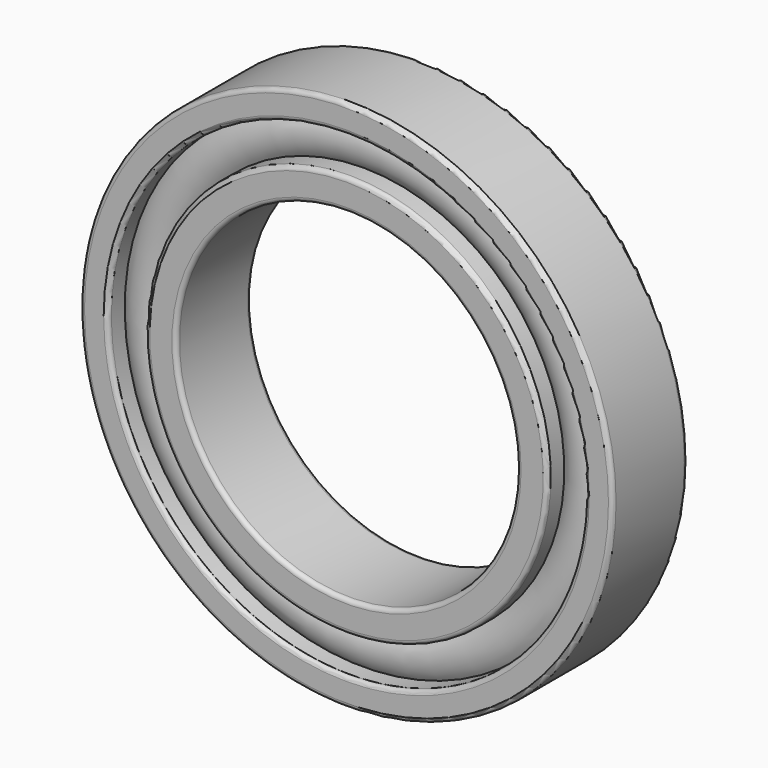
from build123d import *

# Parameters (mm, degrees)
F0_R     = 62.5
F0_R_2   = 40
F1_DEPTH = 11
F4_R     = 1


# Not quite as in the source:
# - a feature names something its author has since deleted; it is built from what else it names


with BuildPart() as f1:
    # F0 (on Front) → F1 (new body, symmetric)
    with BuildSketch(Plane.XZ):
        Circle(F0_R)
        Circle(F0_R_2, mode=Mode.SUBTRACT)
    extrude(amount=F1_DEPTH, both=True)

    # F2 (on Right) → F3 (revolve, cut)
    with BuildSketch(Plane.YZ):
        with BuildLine():
            Line((-6.0737138556, 56), (-21, 56))
            Line((-21, 56), (-21, 47.2))
            Line((-21, 47.2), (-6.0737138556, 47.2))
            ThreePointArc((-6.0737138556, 47.2), (-7.5, 51.6), (-6.0737138556, 56))
        make_face()
        with BuildLine():
            Line((21, 47.2), (21, 56))
            Line((21, 56), (6.0737138556, 56))
            ThreePointArc((6.0737138556, 56), (7.5, 51.6), (6.0737138556, 47.2))
            Line((6.0737138556, 47.2), (21, 47.2))
        make_face()
    revolve(axis=Axis((0, 16.4881043163, 0), (0, 1, 0)), mode=Mode.SUBTRACT)

    # F4
    f4_edges = [f1.edges().sort_by_distance(p)[0] for p in [
        (-62.5, 11, 0),
        (-62.5, -11, 0),
        (-40, 11, 0),
        (-40, -11, 0),
        (0, -11, -56),
        (0, -11, -47.2),
        (0, 11, -56),
        (0, 11, -47.2),
    ]]
    fillet(f4_edges, radius=F4_R)


solid = f1.part
